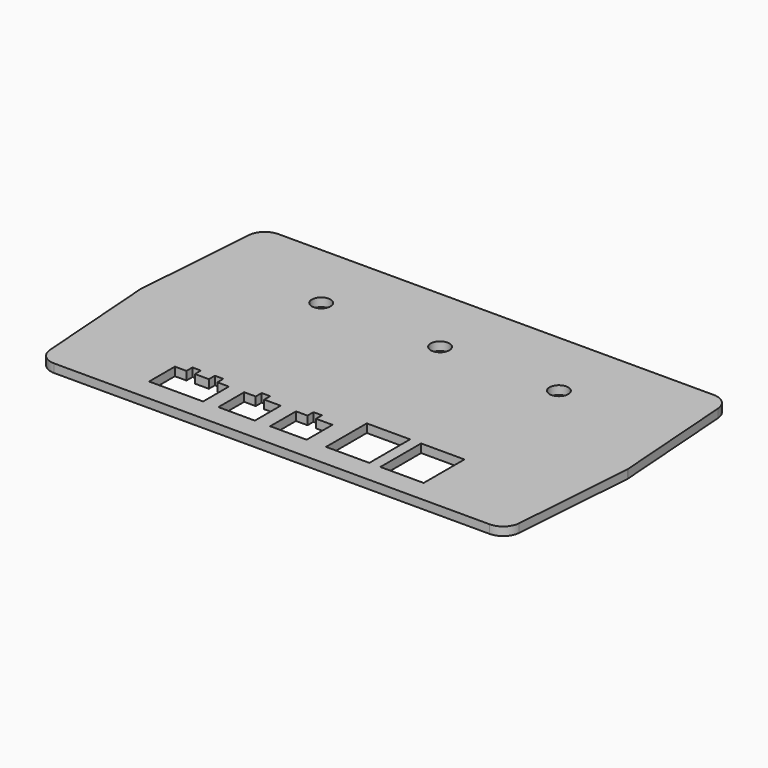
from build123d import *

# Parameters (mm, degrees)
F0_W     = 12.75
F0_H     = 15
F0_R     = 2.75
F1_DEPTH = 2.5
F2_R     = 1.5


with BuildPart() as f1:
    # F0 (on Top) → F1 (new body)
    with BuildSketch(Plane.XY):
        with BuildLine():
            ThreePointArc((69.087259747, 36.6126784789), (67.5053247579, 39.9115155602), (64.1004306622, 41.25))
            Line((64.1004306622, 41.25), (-64.1004306622, 41.25))
            ThreePointArc((-64.1004306622, 41.25), (-67.5053247579, 39.9115155602), (-69.087259747, 36.6126784789))
            Line((-69.087259747, 36.6126784789), (-71.75, 0))
            Line((-71.75, 0), (-69.087259747, -36.6126784789))
            ThreePointArc((-69.087259747, -36.6126784789), (-67.5053247579, -39.9115155602), (-64.1004306622, -41.25))
            Line((-64.1004306622, -41.25), (64.1004306622, -41.25))
            ThreePointArc((64.1004306622, -41.25), (67.5053247579, -39.9115155602), (69.087259747, -36.6126784789))
            Line((69.087259747, -36.6126784789), (71.75, 0))
            Line((71.75, 0), (69.087259747, 36.6126784789))
        make_face()
        Polygon((-25.55, -25.15), (-25.55, -34.65), (-41.45, -34.65), (-41.45, -25.15), (-38.05, -25.15), (-38.05, -22.95), (-35.55, -22.95), (-35.55, -25.15), (-31.45, -25.15), (-31.45, -22.95), (-28.95, -22.95), (-28.95, -25.15), align=None, mode=Mode.SUBTRACT)
        Polygon((-10.3, -25.15), (-10.3, -34.65), (-21.05, -34.65), (-21.05, -25.15), (-17.65, -25.15), (-17.65, -22.95), (-15.15, -22.95), (-15.15, -25.15), align=None, mode=Mode.SUBTRACT)
        Polygon((4.95, -25.15), (4.95, -34.65), (-5.8, -34.65), (-5.8, -25.15), (-2.4, -25.15), (-2.4, -22.95), (0.1, -22.95), (0.1, -25.15), align=None, mode=Mode.SUBTRACT)
        with Locations((17.025, -27.15)):
            Rectangle(F0_W, F0_H, mode=Mode.SUBTRACT)
        with Locations((33.025, -27.15)):
            Rectangle(F0_W, F0_H, mode=Mode.SUBTRACT)
        with Locations((-35, 20.625)):
            Circle(F0_R, mode=Mode.SUBTRACT)
        with Locations((0, 20.625)):
            Circle(F0_R, mode=Mode.SUBTRACT)
        with Locations((35, 20.625)):
            Circle(F0_R, mode=Mode.SUBTRACT)
    extrude(amount=F1_DEPTH)

    # F2
    f2_edges = [f1.edges().sort_by_distance(p)[0] for p in [
        (-71.75, 0, 1.25),
        (71.75, 0, 1.25),
    ]]
    fillet(f2_edges, radius=F2_R)


solid = f1.part
